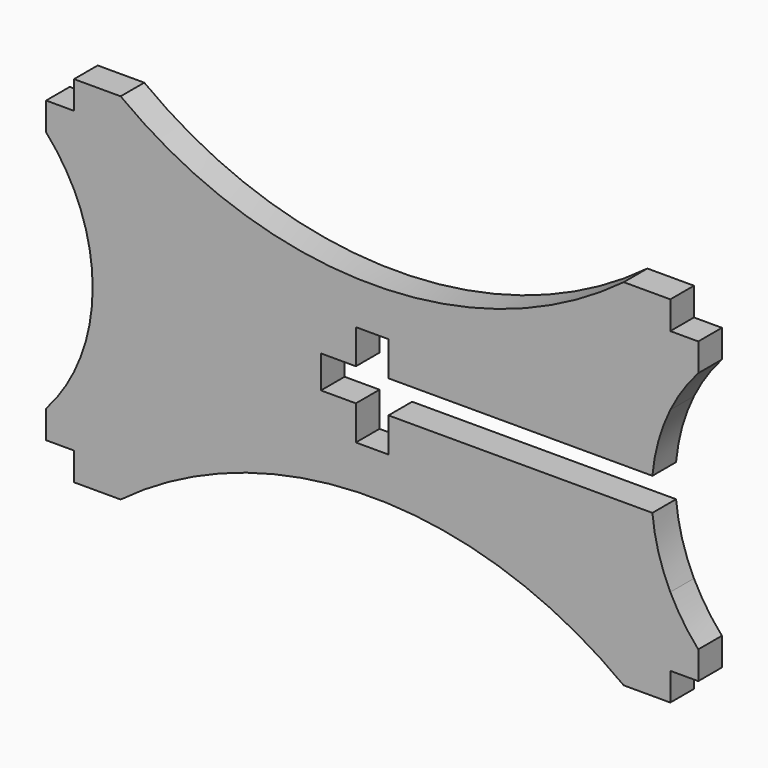
from build123d import *

# Parameters (mm, degrees)
F1_DEPTH = 3.175


# Not quite as in the source:
# - a length typed as a fraction of an inch, garbled in the dataset ("3 / 203.2 mm" for 3/8 in), is restored


with BuildPart() as f1:
    # F0 (on Front) → F1 (new body)
    with BuildSketch(Plane.XZ):
        with BuildLine():
            Line((32, -16.05), (35, -16.05))
            Line((35, -16.05), (35, -13.05))
            ThreePointArc((35, -13.05), (33.3469639854, -10.9330653905), (32, -8.6093553766))
            Line((32, -8.6093553766), (32, -16.05))
        make_face()
        with BuildLine():
            ThreePointArc((32, 8.6093553766), (33.3469639854, 10.9330653905), (35, 13.05))
            Line((35, 13.05), (35, 16.05))
            Line((35, 16.05), (32, 16.05))
            Line((32, 16.05), (32, 8.6093553766))
        make_face()
        with BuildLine():
            Line((-35, -16.05), (-32, -16.05))
            Line((-32, -16.05), (-32, -8.6093553766))
            ThreePointArc((-32, -8.6093553766), (-33.3469639854, -10.9330653905), (-35, -13.05))
            Line((-35, -13.05), (-35, -16.05))
        make_face()
        with BuildLine():
            Line((27, -19.05), (32, -19.05))
            Line((32, -19.05), (32, -16.05))
            Line((32, -16.05), (32, -8.6093553766))
            ThreePointArc((32, -8.6093553766), (30.7239047108, -5.268020684), (30.0785620254, -1.75))
            Line((30.0785620254, -1.75), (1.75, -1.75))
            Line((1.75, -1.75), (1.75, -5.45))
            Line((1.75, -5.45), (-1.75, -5.45))
            Line((-1.75, -5.45), (-1.75, -1.75))
            Line((-1.75, -1.75), (-5.5, -1.75))
            Line((-5.5, -1.75), (-5.5, 0))
            Line((-5.5, 0), (-30, 0))
            ThreePointArc((-30, 0), (-30.5065696236, -4.4193042439), (-32, -8.6093553766))
            Line((-32, -8.6093553766), (-32, -16.05))
            Line((-32, -16.05), (-32, -19.05))
            Line((-32, -19.05), (-27, -19.05))
            ThreePointArc((-27, -19.05), (0, -10.05), (27, -19.05))
        make_face()
        with BuildLine():
            ThreePointArc((30.0785620254, 1.75), (30.7239047108, 5.268020684), (32, 8.6093553766))
            Line((32, 8.6093553766), (32, 16.05))
            Line((32, 16.05), (32, 19.05))
            Line((32, 19.05), (27, 19.05))
            ThreePointArc((27, 19.05), (0, 10.05), (-27, 19.05))
            Line((-27, 19.05), (-32, 19.05))
            Line((-32, 19.05), (-32, 16.05))
            Line((-32, 16.05), (-32, 8.6093553766))
            ThreePointArc((-32, 8.6093553766), (-30.5065696236, 4.4193042439), (-30, 0))
            Line((-30, 0), (-5.5, 0))
            Line((-5.5, 0), (-5.5, 1.75))
            Line((-5.5, 1.75), (-1.75, 1.75))
            Line((-1.75, 1.75), (-1.75, 5.45))
            Line((-1.75, 5.45), (1.75, 5.45))
            Line((1.75, 5.45), (1.75, 1.75))
            Line((1.75, 1.75), (30.0785620254, 1.75))
        make_face()
        with BuildLine():
            ThreePointArc((-35, 13.05), (-33.3469639854, 10.9330653905), (-32, 8.6093553766))
            Line((-32, 8.6093553766), (-32, 16.05))
            Line((-32, 16.05), (-35, 16.05))
            Line((-35, 16.05), (-35, 13.05))
        make_face()
    extrude(amount=F1_DEPTH)


solid = f1.part
